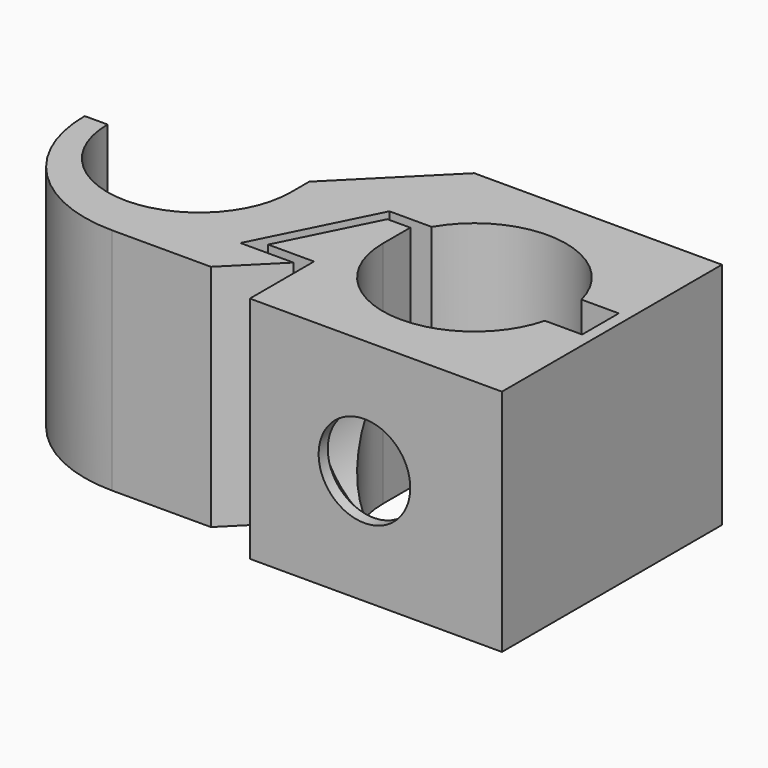
from build123d import *

# Parameters (mm, degrees)
F1_DEPTH = 5
F4_SIZE  = 1.99999
F5_R     = 5.99999
F6_SIZE  = 4


# Not quite as in the source:
# - a fillet or chamfer is up to 0.001 mm smaller than in the source, because OpenCascade refuses the exact size


with BuildPart() as f1:
    # F0 (on Top) → F1 (new body, symmetric)
    with BuildSketch(Plane.XY):
        with BuildLine():
            ThreePointArc((3.8729833462, -1), (-0.5040171699, -3.9681187851), (-4, 0))
            Line((-4, 0), (-4, 1.5))
            Line((-4, 1.5), (-5, 1.5))
            Line((-5, 1.5), (-7, -2.5))
            Line((-7, -2.5), (-5, -2.5))
            Line((-5, -2.5), (-5, -6))
            Line((-5, -6), (6, -6))
            Line((6, -6), (6, 6))
            Line((6, 6), (-8.8090169944, 6))
            Line((-8.8090169944, 6), (-8.8090169944, 1))
            ThreePointArc((-8.8090169944, 1), (-12.8090169944, -3), (-16.8090169944, 1))
            Line((-16.8090169944, 1), (-17.8090169944, 1))
            Line((-17.8090169944, 1), (-17.8090169944, -5))
            Line((-17.8090169944, -5), (-8.8090169944, -5))
            Line((-8.8090169944, -5), (-5.5, -5))
            Line((-5.5, -5), (-5.5, -3))
            Line((-5.5, -3), (-7.8090169944, -3))
            Line((-7.8090169944, -3), (-5.3090169944, 2))
            Line((-5.3090169944, 2), (-3.4641016151, 2))
            ThreePointArc((-3.4641016151, 2), (0.5401815135, 3.9633576589), (3.8729833462, 1))
            Line((3.8729833462, 1), (5.5, 1))
            Line((5.5, 1), (5.5, -1))
            Line((5.5, -1), (3.8729833462, -1))
        make_face()
    extrude(amount=F1_DEPTH, both=True)

    # F2 (on Top) → F3 (revolve, cut)
    with BuildSketch(Plane.XY):
        Polygon((0, 0), (-4, 0), (-4, -3.5), (-2, -5.5), (-2, -6), (0, -6), align=None)
    revolve(axis=Axis((0, -2.25, 0), (0, -1, 0)), mode=Mode.SUBTRACT)

    # F4 (size 2 in the source; OpenCascade refuses exactly that, so slightly less here)
    f4_edges = [f1.edges().sort_by_distance(p)[0] for p in [
        (-5.5, -5, 0),
    ]]
    chamfer(f4_edges, length=F4_SIZE)

    # F5 (radius 6 in the source; OpenCascade refuses exactly that, so slightly less here)
    f5_edges = [f1.edges().sort_by_distance(p)[0] for p in [
        (-17.809017, -5, 0),
    ]]
    fillet(f5_edges, radius=F5_R)

    # F6
    f6_edges = [f1.edges().sort_by_distance(p)[0] for p in [
        (-8.809017, 6, 0),
    ]]
    chamfer(f6_edges, length=F6_SIZE)


solid = f1.part
